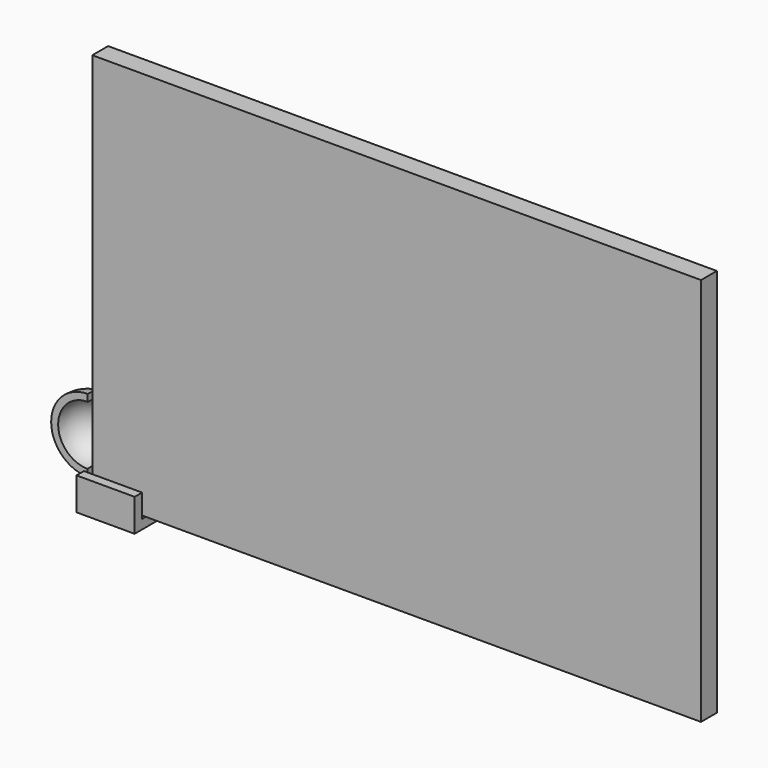
from build123d import *

# Parameters (mm, degrees)
F0_W     = 261.8
F0_H     = 167.3
F1_DEPTH = 8.5
F3_ANGLE = 90
F5_DEPTH = 25


with BuildPart() as f1:
    # F0 (on Front) → F1 (new body)
    with BuildSketch(Plane.XZ):
        with Locations((130.9, 83.65)):
            Rectangle(F0_W, F0_H)
    extrude(amount=F1_DEPTH)


with BuildPart() as f3:
    # F2 (on face) → F3 (revolve)
    with BuildSketch(Plane.XZ.offset(8.5)):
        with BuildLine():
            Line((-2, 35.4), (-2, 38.4))
            ThreePointArc((-2, 38.4), (-17.7, 22.7), (-2, 7))
            Line((-2, 7), (-2, 10))
            ThreePointArc((-2, 10), (-14.7, 22.7), (-2, 35.4))
        make_face()
    revolve(axis=Axis((-2, -8.5, 29.05), (0, 0, -1)), revolution_arc=F3_ANGLE)

    # F4 (on face) → F5 (join)
    with BuildSketch(Plane.YZ.offset(-2)):
        Polygon((6, 38.4), (2, 38.4), (2, 0), (-10.5, 0), (-10.5, 10), (-14.5, 10), (-14.5, -4), (6, -4), align=None)
    extrude(amount=F5_DEPTH)


solid = Compound([f1.part, f3.part])
